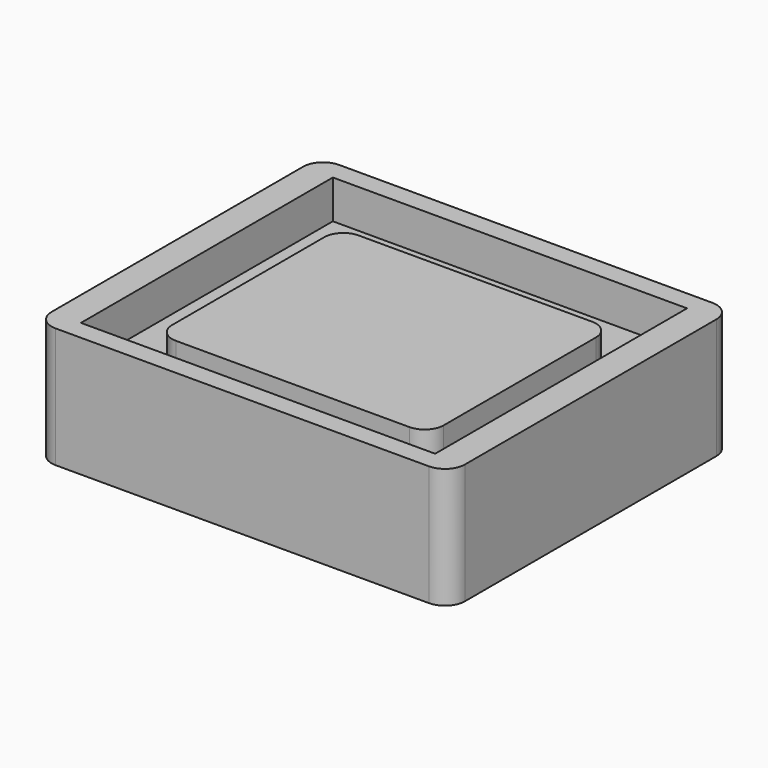
from build123d import *

# Parameters (mm, degrees)
F0_W     = 105
F0_H     = 90
F0_W_2   = 90
F0_H_2   = 80
F1_DEPTH = 15.3
F2_R     = 5.069848481
F0_W_3   = 69
F0_H_3   = 58
F3_DEPTH = 5.5
F4_DEPTH = 11.8
F5_R     = 4.8284271247


with BuildPart() as f1:
    # F0 (on Top) → F1 (new body, symmetric)
    with BuildSketch(Plane.XY):
        Rectangle(F0_W, F0_H)
        Rectangle(F0_W_2, F0_H_2, mode=Mode.SUBTRACT)
    extrude(amount=F1_DEPTH, both=True)

    # F2
    f2_edges = [f1.edges().sort_by_distance(p)[0] for p in [
        (52.5, -45, 0),
        (-52.5, -45, 0),
        (-52.5, 45, 0),
        (52.5, 45, 0),
    ]]
    fillet(f2_edges, radius=F2_R)

    # F0 (on Top) → F3 (join)
    with BuildSketch(Plane.XY):
        Rectangle(F0_W_2, F0_H_2)
        Rectangle(F0_W_3, F0_H_3, mode=Mode.SUBTRACT)
    extrude(amount=F3_DEPTH)

    # F0 (on Top) → F4 (join)
    with BuildSketch(Plane.XY):
        Rectangle(F0_W_3, F0_H_3)
    extrude(amount=F4_DEPTH)

    # F5
    f5_edges = [f1.edges().sort_by_distance(p)[0] for p in [
        (34.5, -29, 8.65),
        (34.5, 29, 8.65),
        (-34.5, 29, 8.65),
        (-34.5, -29, 8.65),
    ]]
    fillet(f5_edges, radius=F5_R)


solid = f1.part
